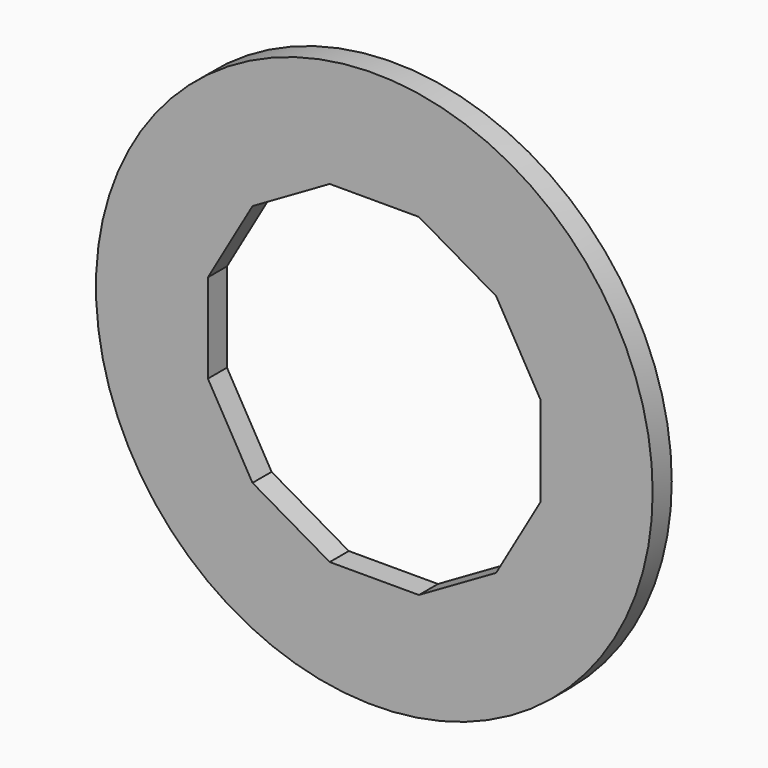
from build123d import *

# Parameters (mm, degrees)
F0_R     = 70
F1_DEPTH = 3


# Not quite as in the source:
# - a feature of the source that left no trace in its solid (it failed there, or was rolled back) is left out


with BuildPart() as f1:
    # F0 (on Front) → F1 (new body, symmetric)
    with BuildSketch(Plane.XZ):
        Circle(F0_R)
        Polygon((-30.6363262968, 30.6363262968), (-11.2136737032, 41.85), (11.2136737032, 41.85), (30.6363262968, 30.6363262968), (41.85, 11.2136737032), (41.85, -11.2136737032), (30.6363262968, -30.6363262968), (11.2136737032, -41.85), (-11.2136737032, -41.85), (-30.6363262968, -30.6363262968), (-41.85, -11.2136737032), (-41.85, 11.2136737032), align=None, mode=Mode.SUBTRACT)
    extrude(amount=F1_DEPTH, both=True)


solid = f1.part
